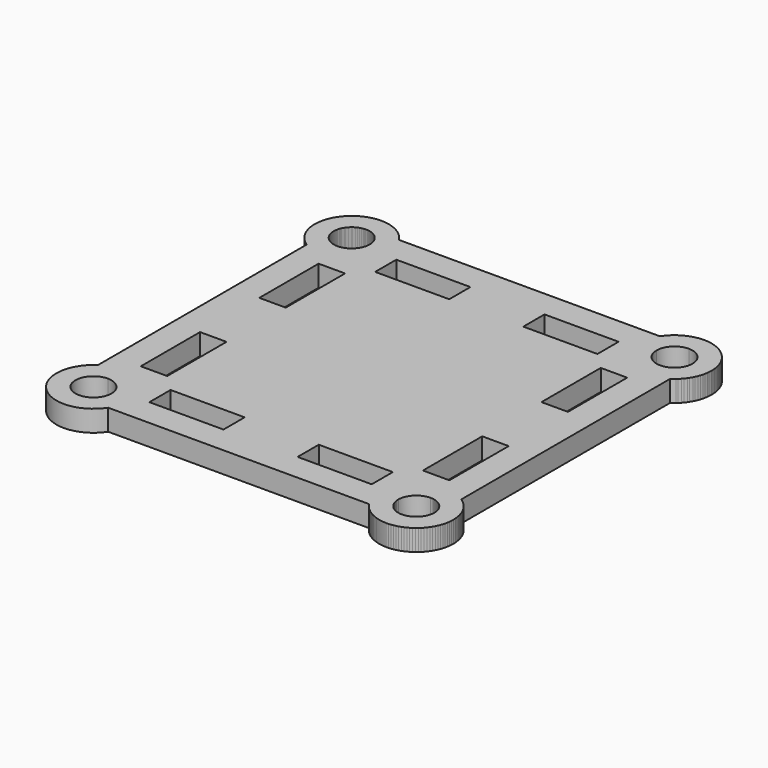
from build123d import *

# Parameters (mm, degrees)
F2_DEPTH  = 2
F4_ANGLE  = 45
F8_R      = 1.7
F9_DEPTH  = 2.001
F10_W     = 7
F10_H     = 1.25
F11_DEPTH = 2.001
F12_ANGLE = 90
F13_W     = 7
F13_H     = 2.5
F13_W_2   = 2.5
F13_H_2   = 7
F14_DEPTH = 2.001


# Not quite as in the source:
# - a feature names something its author has since deleted; it is built from what else it names


with BuildPart() as f2:
    # F1 (on Top) → F2 (new body)
    with BuildSketch(Plane.XY):
        with BuildLine():
            ThreePointArc((-12.3236370697, 17.17), (-17.7248737342, 17.7248737342), (-17.17, 12.3236370697))
            ThreePointArc((-17.17, 12.3236370697), (-16.2519305724, 11.8964742243), (-15.25, 11.75))
            Line((-15.25, 11.75), (-15.25, 13.55))
            ThreePointArc((-15.25, 13.55), (-16.452081528, 16.452081528), (-13.55, 15.25))
            Line((-13.55, 15.25), (-11.75, 15.25))
            ThreePointArc((-11.75, 15.25), (-11.8964742243, 16.2519305724), (-12.3236370697, 17.17))
        make_face()
        with BuildLine():
            ThreePointArc((-15.25, 11.75), (-14.2480694276, 11.8964742243), (-13.33, 12.3236370697))
            ThreePointArc((-13.33, 12.3236370697), (-12.7751262658, 12.7751262658), (-12.3236370697, 13.33))
            ThreePointArc((-12.3236370697, 13.33), (-11.8964742243, 14.2480694276), (-11.75, 15.25))
            Line((-11.75, 15.25), (-13.55, 15.25))
            ThreePointArc((-13.55, 15.25), (-14.047918472, 14.047918472), (-15.25, 13.55))
            Line((-15.25, 13.55), (-15.25, 11.75))
        make_face()
        with BuildLine():
            Line((15.25, 13.55), (15.25, 11.75))
            ThreePointArc((15.25, 11.75), (16.2519305724, 11.8964742243), (17.17, 12.3236370697))
            ThreePointArc((17.17, 12.3236370697), (18.3297727189, 13.5871710852), (18.75, 15.25))
            ThreePointArc((18.75, 15.25), (16.2519305724, 18.6035257757), (12.3236370697, 17.17))
            ThreePointArc((12.3236370697, 17.17), (11.8964742243, 16.2519305724), (11.75, 15.25))
            Line((11.75, 15.25), (13.55, 15.25))
            ThreePointArc((13.55, 15.25), (15.25, 16.95), (16.95, 15.25))
            ThreePointArc((16.95, 15.25), (16.452081528, 14.047918472), (15.25, 13.55))
        make_face()
        with BuildLine():
            ThreePointArc((12.3236370697, 13.33), (12.7751262658, 12.7751262658), (13.33, 12.3236370697))
            ThreePointArc((13.33, 12.3236370697), (14.2480694276, 11.8964742243), (15.25, 11.75))
            Line((15.25, 11.75), (15.25, 13.55))
            ThreePointArc((15.25, 13.55), (14.047918472, 14.047918472), (13.55, 15.25))
            Line((13.55, 15.25), (11.75, 15.25))
            ThreePointArc((11.75, 15.25), (11.8964742243, 14.2480694276), (12.3236370697, 13.33))
        make_face()
        with BuildLine():
            Line((13.33, 12.3236370697), (13.33, -12.3236370697))
            ThreePointArc((13.33, -12.3236370697), (14.2480694276, -11.8964742243), (15.25, -11.75))
            Line((15.25, -11.75), (15.25, 11.75))
            ThreePointArc((15.25, 11.75), (14.2480694276, 11.8964742243), (13.33, 12.3236370697))
        make_face()
        with BuildLine():
            ThreePointArc((-11.75, 15.25), (-11.8964742243, 14.2480694276), (-12.3236370697, 13.33))
            Line((-12.3236370697, 13.33), (12.3236370697, 13.33))
            ThreePointArc((12.3236370697, 13.33), (11.8964742243, 14.2480694276), (11.75, 15.25))
            Line((11.75, 15.25), (-11.75, 15.25))
        make_face()
        with BuildLine():
            ThreePointArc((-15.25, -11.75), (-14.2480694276, -11.8964742243), (-13.33, -12.3236370697))
            Line((-13.33, -12.3236370697), (-13.33, 12.3236370697))
            ThreePointArc((-13.33, 12.3236370697), (-14.2480694276, 11.8964742243), (-15.25, 11.75))
            Line((-15.25, 11.75), (-15.25, -11.75))
        make_face()
        with BuildLine():
            Line((-17.17, 12.3236370697), (-17.17, -12.3236370697))
            ThreePointArc((-17.17, -12.3236370697), (-16.2519305724, -11.8964742243), (-15.25, -11.75))
            Line((-15.25, -11.75), (-15.25, 11.75))
            ThreePointArc((-15.25, 11.75), (-16.2519305724, 11.8964742243), (-17.17, 12.3236370697))
        make_face()
        with BuildLine():
            Line((15.25, 11.75), (15.25, -11.75))
            ThreePointArc((15.25, -11.75), (16.2519305724, -11.8964742243), (17.17, -12.3236370697))
            Line((17.17, -12.3236370697), (17.17, 12.3236370697))
            ThreePointArc((17.17, 12.3236370697), (16.2519305724, 11.8964742243), (15.25, 11.75))
        make_face()
        with BuildLine():
            ThreePointArc((-12.3236370697, -13.33), (-11.8964742243, -14.2480694276), (-11.75, -15.25))
            Line((-11.75, -15.25), (11.75, -15.25))
            ThreePointArc((11.75, -15.25), (11.8964742243, -14.2480694276), (12.3236370697, -13.33))
            Line((12.3236370697, -13.33), (-12.3236370697, -13.33))
        make_face()
        with BuildLine():
            Line((11.75, -15.25), (-11.75, -15.25))
            ThreePointArc((-11.75, -15.25), (-11.8964742243, -16.2519305724), (-12.3236370697, -17.17))
            Line((-12.3236370697, -17.17), (12.3236370697, -17.17))
            ThreePointArc((12.3236370697, -17.17), (11.8964742243, -16.2519305724), (11.75, -15.25))
        make_face()
        with BuildLine():
            Line((12.3236370697, 17.17), (-12.3236370697, 17.17))
            ThreePointArc((-12.3236370697, 17.17), (-11.8964742243, 16.2519305724), (-11.75, 15.25))
            Line((-11.75, 15.25), (11.75, 15.25))
            ThreePointArc((11.75, 15.25), (11.8964742243, 16.2519305724), (12.3236370697, 17.17))
        make_face()
        with BuildLine():
            ThreePointArc((-12.3236370697, -17.17), (-11.8964742243, -16.2519305724), (-11.75, -15.25))
            Line((-11.75, -15.25), (-13.55, -15.25))
            ThreePointArc((-13.55, -15.25), (-16.452081528, -16.452081528), (-15.25, -13.55))
            Line((-15.25, -13.55), (-15.25, -11.75))
            ThreePointArc((-15.25, -11.75), (-16.2519305724, -11.8964742243), (-17.17, -12.3236370697))
            ThreePointArc((-17.17, -12.3236370697), (-17.7248737342, -17.7248737342), (-12.3236370697, -17.17))
        make_face()
        with BuildLine():
            Line((-13.55, -15.25), (-11.75, -15.25))
            ThreePointArc((-11.75, -15.25), (-11.8964742243, -14.2480694276), (-12.3236370697, -13.33))
            ThreePointArc((-12.3236370697, -13.33), (-12.7751262658, -12.7751262658), (-13.33, -12.3236370697))
            ThreePointArc((-13.33, -12.3236370697), (-14.2480694276, -11.8964742243), (-15.25, -11.75))
            Line((-15.25, -11.75), (-15.25, -13.55))
            ThreePointArc((-15.25, -13.55), (-14.047918472, -14.047918472), (-13.55, -15.25))
        make_face()
        with BuildLine():
            ThreePointArc((12.3236370697, -13.33), (11.8964742243, -14.2480694276), (11.75, -15.25))
            Line((11.75, -15.25), (13.55, -15.25))
            ThreePointArc((13.55, -15.25), (14.047918472, -14.047918472), (15.25, -13.55))
            Line((15.25, -13.55), (15.25, -11.75))
            ThreePointArc((15.25, -11.75), (14.2480694276, -11.8964742243), (13.33, -12.3236370697))
            ThreePointArc((13.33, -12.3236370697), (12.7751262658, -12.7751262658), (12.3236370697, -13.33))
        make_face()
        with BuildLine():
            Line((13.55, -15.25), (11.75, -15.25))
            ThreePointArc((11.75, -15.25), (11.8964742243, -16.2519305724), (12.3236370697, -17.17))
            ThreePointArc((12.3236370697, -17.17), (16.2519305724, -18.6035257757), (18.75, -15.25))
            ThreePointArc((18.75, -15.25), (18.3297727189, -13.5871710852), (17.17, -12.3236370697))
            ThreePointArc((17.17, -12.3236370697), (16.2519305724, -11.8964742243), (15.25, -11.75))
            Line((15.25, -11.75), (15.25, -13.55))
            ThreePointArc((15.25, -13.55), (16.452081528, -14.047918472), (16.95, -15.25))
            ThreePointArc((16.95, -15.25), (15.25, -16.95), (13.55, -15.25))
        make_face()
        with BuildLine():
            ThreePointArc((-13.33, -12.3236370697), (-12.7751262658, -12.7751262658), (-12.3236370697, -13.33))
            Line((-12.3236370697, -13.33), (12.3236370697, -13.33))
            ThreePointArc((12.3236370697, -13.33), (12.7751262658, -12.7751262658), (13.33, -12.3236370697))
            Line((13.33, -12.3236370697), (13.33, 12.3236370697))
            ThreePointArc((13.33, 12.3236370697), (12.7751262658, 12.7751262658), (12.3236370697, 13.33))
            Line((12.3236370697, 13.33), (-12.3236370697, 13.33))
            ThreePointArc((-12.3236370697, 13.33), (-12.7751262658, 12.7751262658), (-13.33, 12.3236370697))
            Line((-13.33, 12.3236370697), (-13.33, -12.3236370697))
        make_face()
    extrude(amount=F2_DEPTH)


with BuildPart() as f4_1:
    # F4: copy of F2
    add(f2.part.rotate(Axis((0, 0, 43.582893908), (0, 0, 1)), F4_ANGLE))


with BuildPart() as f2_1:
    add(f2.part)

    # F5: union F4_1
    add(f4_1.part)

    # F8 (on face) → F9 (cut, through all)
    with BuildSketch(Plane.XY.offset(2)):
        with BuildLine():
            Line((-3.4268960921, 20.8551507738), (-7.1120468659, 17.17))
            Line((-7.1120468659, 17.17), (7.1120468659, 17.17))
            Line((7.1120468659, 17.17), (3.4268960921, 20.8551507738))
            ThreePointArc((3.4268960921, 20.8551507738), (0, 25.0667568262), (-3.4268960921, 20.8551507738))
        make_face()
        with Locations((0, 21.5667568262)):
            Circle(F8_R, mode=Mode.SUBTRACT)
        with BuildLine():
            Line((20.8551507738, 3.4268960921), (17.17, 7.1120468659))
            Line((17.17, 7.1120468659), (17.17, -7.1120468659))
            Line((17.17, -7.1120468659), (20.8551507738, -3.4268960921))
            ThreePointArc((20.8551507738, -3.4268960921), (25.0667568262, 0), (20.8551507738, 3.4268960921))
        make_face()
        with Locations((21.5667568262, 0)):
            Circle(F8_R, mode=Mode.SUBTRACT)
        with BuildLine():
            Line((7.1120468659, -17.17), (-7.1120468659, -17.17))
            Line((-7.1120468659, -17.17), (-3.4268960921, -20.8551507738))
            ThreePointArc((-3.4268960921, -20.8551507738), (0, -25.0667568262), (3.4268960921, -20.8551507738))
            Line((3.4268960921, -20.8551507738), (7.1120468659, -17.17))
        make_face()
        with Locations((0, -21.5667568262)):
            Circle(F8_R, mode=Mode.SUBTRACT)
        with BuildLine():
            Line((-17.17, -7.1120468659), (-17.17, 7.1120468659))
            Line((-17.17, 7.1120468659), (-20.8551507738, 3.4268960921))
            ThreePointArc((-20.8551507738, 3.4268960921), (-25.0667568262, 0), (-20.8551507738, -3.4268960921))
            Line((-20.8551507738, -3.4268960921), (-17.17, -7.1120468659))
        make_face()
        with Locations((-21.5667568262, 0)):
            Circle(F8_R, mode=Mode.SUBTRACT)
    extrude(amount=-F9_DEPTH, mode=Mode.SUBTRACT)

    # F10 (on face) → F11 (cut, through all)
    with BuildSketch(Plane.XY.offset(2)):
        Polygon((-9.3647099602, 12.08), (-3.5, 12.08), (-3.5, 13.33), (-10.5, 13.33), (-10.5, 13.2152900398), align=None)
        Polygon((-10.5, 12.08), (-9.3647099602, 12.08), (-10.5, 13.2152900398), align=None)
        with Locations((-7, 13.955)):
            Rectangle(F10_W, F10_H)
        Polygon((10.5, 13.33), (3.5, 13.33), (3.5, 12.08), (9.3647099602, 12.08), (10.5, 13.2152900398), align=None)
        with Locations((7, 13.955)):
            Rectangle(F10_W, F10_H)
        Polygon((10.5, -13.2152900398), (10.5, -12.08), (9.3647099602, -12.08), align=None)
        Polygon((10.5, -13.33), (10.5, -13.2152900398), (9.3647099602, -12.08), (3.5, -12.08), (3.5, -13.33), align=None)
        with Locations((7, -13.955)):
            Rectangle(F10_W, F10_H)
        Polygon((-10.5, -13.33), (-3.5, -13.33), (-3.5, -12.08), (-9.3647099602, -12.08), (-10.5, -13.2152900398), align=None)
        with Locations((-7, -13.955)):
            Rectangle(F10_W, F10_H)
        Polygon((-10.5, -13.2152900398), (-9.3647099602, -12.08), (-10.5, -12.08), align=None)
    extrude(amount=-F11_DEPTH, mode=Mode.SUBTRACT)


with BuildPart() as f12_1:
    # F12: copy of F2
    add(f2_1.part.rotate(Axis((0, 0, 43.582893908), (0, 0, 1)), F12_ANGLE))


with BuildPart() as f14_tool:
    # F13 (on face) → F14 (new body, through all)
    with BuildSketch(Plane.XY.offset(2)):
        with Locations((-7, 13.33)):
            Rectangle(F13_W, F13_H)
        with Locations((-13.33, 7)):
            Rectangle(F13_W_2, F13_H_2)
        with Locations((7, 13.33)):
            Rectangle(F13_W, F13_H)
        with Locations((13.33, 7)):
            Rectangle(F13_W_2, F13_H_2)
        with Locations((-13.33, -7)):
            Rectangle(F13_W_2, F13_H_2)
        with Locations((13.33, -7)):
            Rectangle(F13_W_2, F13_H_2)
        with Locations((7, -13.33)):
            Rectangle(F13_W, F13_H)
        with Locations((-7, -13.33)):
            Rectangle(F13_W, F13_H)
    extrude(amount=-F14_DEPTH)


with BuildPart() as f2_2:
    add(f2_1.part)

    # F14: cut by f14_tool
    add(f14_tool.part, mode=Mode.SUBTRACT)


with BuildPart() as f12_1_1:
    add(f12_1.part)

    # F14: cut by f14_tool
    add(f14_tool.part, mode=Mode.SUBTRACT)


solid = Compound([f2_2.part, f12_1_1.part])
